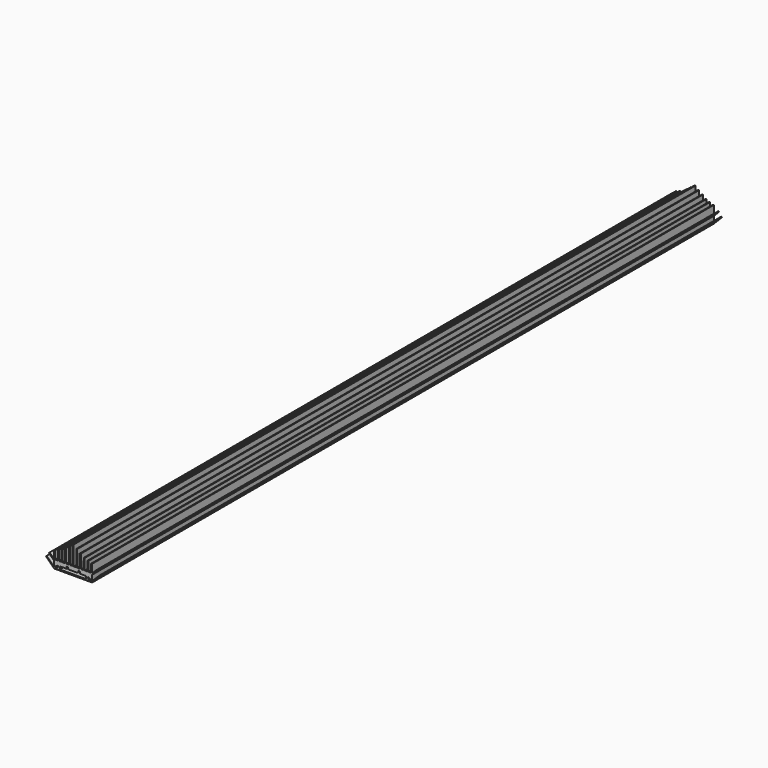
from build123d import *

# Parameters (mm, degrees)
F1_DEPTH = 1420
F3_DEPTH = 1420
F5_DEPTH = 1420


with BuildPart() as f1:
    # F0 (on Front) → F1 (new body)
    with BuildSketch(Plane.XZ):
        with BuildLine():
            Line((-32.7227568555, 3.4999999998), (-32.9727568555, 18.4999999998))
            Line((-32.9727568555, 18.4999999998), (-34.4727568555, 18.4999999998))
            Line((-34.4727568555, 18.4999999998), (-34.7227568555, 3.4999999998))
            Line((-34.7227568555, 3.4999999998), (-34.7227568555, -11.5000000002))
            Line((-34.7227568555, -11.5000000002), (-27.5528838745, -11.5000000002))
            Line((-27.5528838745, -11.5000000002), (-27.5528838745, -7.5000000002))
            Line((-27.5528838745, -7.5000000002), (-28.5528838745, -7.5000000002))
            Line((-28.5528838745, -7.5000000002), (-28.5528838745, -9.0000000002))
            Line((-28.5528838745, -9.0000000002), (-32.0528838745, -9.0000000002))
            Line((-32.0528838745, -9.0000000002), (-32.0528838745, -7.0000000002))
            Line((-32.0528838745, -7.0000000002), (-27.7227568555, -4.5000000002))
            Line((-27.7227568555, -4.5000000002), (-27.1091535687, -4.5000000002))
            Line((-27.1091535687, -4.5000000002), (-25.3028838745, -4.5000000002))
            Line((-25.3028838745, -4.5000000002), (-25.3028838745, -9.5000000002))
            Line((-25.3028838745, -9.5000000002), (-23.8028838745, -9.5000000002))
            Line((-23.8028838745, -9.5000000002), (-23.8028838745, -4.5000000002))
            Line((-23.8028838745, -4.5000000002), (-11.2141814145, -4.5000000002))
            Line((-11.2141814145, -4.5000000002), (-12.1783628291, -3.3509333355))
            Line((-12.1783628291, -3.3509333355), (-12.1783628291, -1.4518666708))
            ThreePointArc((-12.1783628291, -1.4518666708), (-10.9283628291, -0.2018666708), (-9.6783628291, -1.4518666708))
            Line((-9.6783628291, -1.4518666708), (-9.6783628291, -2.2018666708))
            Line((-9.6783628291, -2.2018666708), (-7.75, -4.5000000002))
            Line((-7.75, -4.5000000002), (0, -4.5000000002))
            Line((0, -4.5000000002), (0, 38.4999999998))
            Line((0, 38.4999999998), (-0.75, 38.4999999998))
            Line((-0.75, 38.4999999998), (-1, 3.4999999998))
            Line((-1, 3.4999999998), (-5.75, 3.4999999998))
            Line((-5.75, 3.4999999998), (-6, 33.4999999998))
            Line((-6, 33.4999999998), (-7.5, 33.4999999998))
            Line((-7.5, 33.4999999998), (-7.75, 3.4999999998))
            Line((-7.75, 3.4999999998), (-12.6212390675, 3.4999999998))
            Line((-12.6212390675, 3.4999999998), (-12.8712390675, 28.4999999998))
            Line((-12.8712390675, 28.4999999998), (-14.3712390675, 28.4999999998))
            Line((-14.3712390675, 28.4999999998), (-14.6212390675, 3.5015064141))
            Line((-14.6212390675, 3.5015064141), (-19.2384126596, 3.4999999998))
            Line((-19.2384126596, 3.4999999998), (-19.4884126596, 23.4999999998))
            Line((-19.4884126596, 23.4999999998), (-20.9884126596, 23.4999999998))
            Line((-20.9884126596, 23.4999999998), (-21.2384126596, 3.4999999998))
            Line((-21.2384126596, 3.4999999998), (-26, 3.4999999998))
            Line((-26, 3.4999999998), (-26.25, 20.9999999998))
            Line((-26.25, 20.9999999998), (-27.75, 20.9999999998))
            Line((-27.75, 20.9999999998), (-28, 3.4999999998))
            Line((-28, 3.4999999998), (-32.7227568555, 3.4999999998))
        make_face()
    extrude(amount=F1_DEPTH)

    # F2 (on face) → F3 (join)
    with BuildSketch(Plane.XZ.offset(1420)):
        Polygon((-44.0919217063, 10.5585046788), (-34.7227568555, 0.9999999998), (-34.7227568555, 3.4999999998), (-43.0312615345, 11.6191648506), align=None)
        Polygon((-49.3952225652, 3.3618055377), (-34.7227568555, -11.5000000002), (-34.7227568555, -9.0000000002), (-48.3345623934, 4.4224657095), align=None)
    extrude(amount=-F3_DEPTH)

    # F6: F1 across face


with BuildPart() as f5:
    # F4 (on face) → F5 (new body)
    with BuildSketch(Plane.XZ.offset(1420)):
        Polygon((-25.3028838745, -9.5000000002), (-25.3028838745, -4.5000000002), (-27.3028838745, -4.5000000002), (-27.3028838745, -11.5000000002), (0, -11.5000000002), (0, -9.5000000002), align=None)
    extrude(amount=-F5_DEPTH)

    # F7: F5 across face


with BuildPart() as f1_1:
    add(f1.part)
    add(f1.part.mirror(Plane(origin=(0, -710, 16.9999999998), x_dir=(0, 1, 0), z_dir=(1, 0, 0))))


with BuildPart() as f5_1:
    add(f5.part)
    add(f5.part.mirror(Plane(origin=(0, -710, -10.5000000002), x_dir=(0, 1, 0), z_dir=(1, 0, 0))))


solid = Compound([f1_1.part, f5_1.part])
